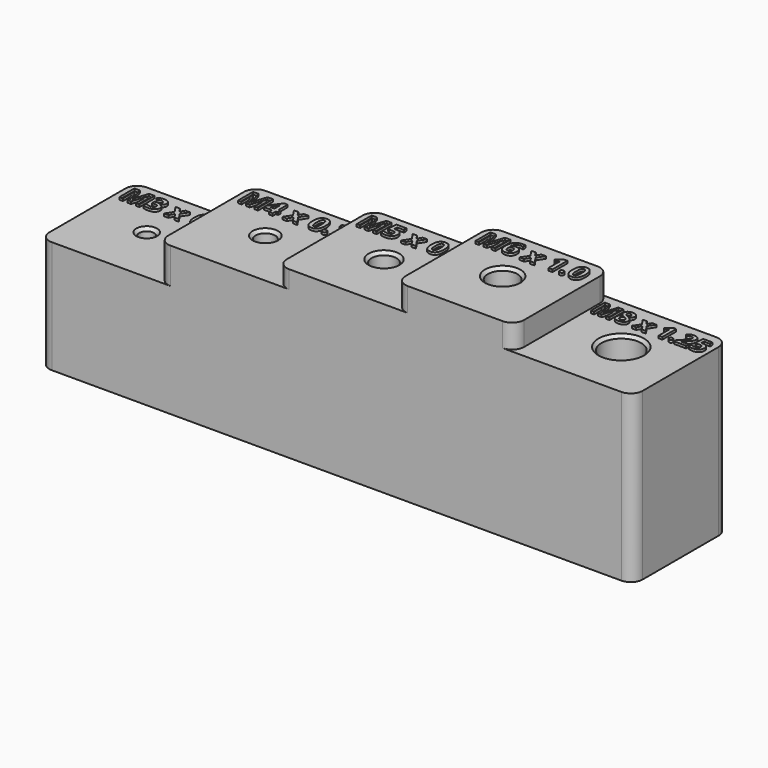
from build123d import *

# Parameters (mm, degrees)
F1_DEPTH      = 20
F3_R          = 1.25
F3_R_2        = 1.65
F3_R_3        = 2.1
F3_R_4        = 2.5
F3_R_5        = 3.35
F4_DEPTH      = 28.001
F5_TEXT_SIZE  = 4.4355459726
F6_DEPTH      = 0.4
F7_TEXT_SIZE  = 4.4212465459
F8_DEPTH      = 0.4
F9_TEXT_SIZE  = 4.4244728655
F10_DEPTH     = 0.4
F11_TEXT_SIZE = 4.4254926818
F12_DEPTH     = 0.4
F13_TEXT_SIZE = 4.1046413502
F14_DEPTH     = 0.4
F15_SIZE      = 0.5
F16_R         = 2


# Not quite as in the source:
# - Text() gives the source's letters only with a copy of the font that has no kerning and outlines rounded to 1/6400 em; it was checked with that copy


with BuildPart() as f1:
    # F0 (on Front) → F1 (new body)
    with BuildSketch(Plane.XZ):
        Polygon((0, 19), (0, 0), (100, 0), (100, 28), (80, 28), (80, 32), (60, 32), (60, 28), (40, 28), (40, 25), (20, 25), (20, 19), align=None)
    extrude(amount=F1_DEPTH)

    # F3 (on offset) → F4 (cut, through all)
    with BuildSketch(Plane(origin=(0, 0, 4), x_dir=(1, 0, 0), z_dir=(0, 0, -1))):
        with Locations((10, 10)):
            Circle(F3_R)
        with Locations((30, 10)):
            Circle(F3_R_2)
        with Locations((50, 10)):
            Circle(F3_R_3)
        with Locations((70, 10)):
            Circle(F3_R_4)
        with Locations((90, 10)):
            Circle(F3_R_5)
    extrude(amount=-F4_DEPTH, mode=Mode.SUBTRACT)

    # F5 (on face) → F6 (join)
    with BuildSketch(Plane.XY.offset(19)):
        with Locations((1, -5)):
            Text('M3 x 0.5', F5_TEXT_SIZE, font='Open Sans', font_style=FontStyle.BOLD, text_align=(TextAlign.LEFT, TextAlign.BOTTOM))
    extrude(amount=F6_DEPTH)

    # F7 (on face) → F8 (join)
    with BuildSketch(Plane.XY.offset(25)):
        with Locations((21, -5)):
            Text('M4 x 0.7', F7_TEXT_SIZE, font='Open Sans', font_style=FontStyle.BOLD, text_align=(TextAlign.LEFT, TextAlign.BOTTOM))
    extrude(amount=F8_DEPTH)

    # F9 (on face) → F10 (join)
    with BuildSketch(Plane.XY.offset(28)):
        with Locations((41, -5)):
            Text('M5 x 0.8', F9_TEXT_SIZE, font='Open Sans', font_style=FontStyle.BOLD, text_align=(TextAlign.LEFT, TextAlign.BOTTOM))
    extrude(amount=F10_DEPTH)

    # F11 (on face) → F12 (join)
    with BuildSketch(Plane.XY.offset(32)):
        with Locations((61, -5)):
            Text('M6 x 1.0', F11_TEXT_SIZE, font='Open Sans', font_style=FontStyle.BOLD, text_align=(TextAlign.LEFT, TextAlign.BOTTOM))
    extrude(amount=F12_DEPTH)

    # F13 (on face) → F14 (join)
    with BuildSketch(Plane.XY.offset(28)):
        with Locations((80.5, -5)):
            Text('M8 x 1.25', F13_TEXT_SIZE, font='Open Sans', font_style=FontStyle.BOLD, text_align=(TextAlign.LEFT, TextAlign.BOTTOM))
    extrude(amount=F14_DEPTH)

    # F15
    f15_edges = [f1.edges().sort_by_distance(p)[0] for p in [
        (8.75, -10, 19),
        (28.35, -10, 25),
        (47.9, -10, 28),
        (67.5, -10, 32),
        (86.65, -10, 28),
    ]]
    chamfer(f15_edges, length=F15_SIZE)

    # F16
    f16_edges = [f1.edges().sort_by_distance(p)[0] for p in [
        (0, -20, 9.5),
        (0, 0, 9.5),
        (20, -20, 22),
        (20, 0, 22),
        (40, 0, 26.5),
        (40, -20, 26.5),
        (60, -20, 30),
        (60, 0, 30),
        (80, -20, 30),
        (80, 0, 30),
        (100, 0, 14),
        (100, -20, 14),
    ]]
    fillet(f16_edges, radius=F16_R)


solid = f1.part
